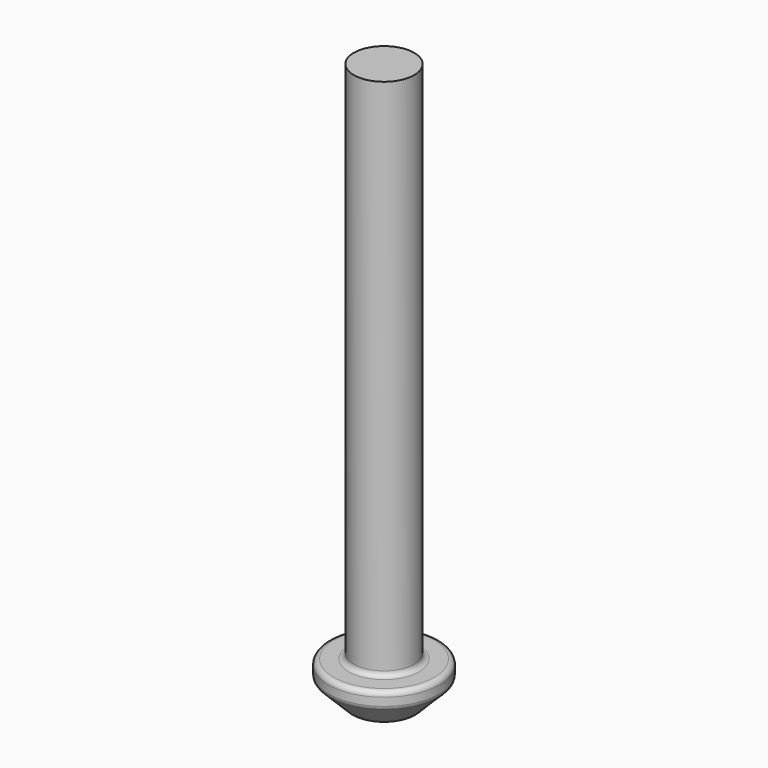
from build123d import *

# Parameters (mm, degrees)
F1_R     = 2.75
F1_R_2   = 1.5
F2_DEPTH = 2
F3_START = 1.5
F3_DEPTH = 0.5
F4_START = 2
F4_DEPTH = 26
F5_SIZE2 = 1.25
F5_SIZE  = 1.25
F6_R     = 0.25


# Not quite as in the source:
# - a feature names something its author has since deleted; it is built from what else it names


with BuildPart() as f2:
    # F1 (on Top) → F2 (new body)
    with BuildSketch(Plane.XY):
        Circle(F1_R)
        Circle(F1_R_2, mode=Mode.SUBTRACT)
        Circle(F1_R_2)
        Polygon((-0.5773502692, -1), (-1.1547005384, 0), (-0.5773502692, 1), (0.5773502692, 1), (1.1547005384, 0), (0.5773502692, -1), align=None, mode=Mode.SUBTRACT)
    extrude(amount=F2_DEPTH)

    # F1 (on Top) → F3 (join)
    with BuildSketch(Plane.XY.offset(F3_START)):
        Polygon((-0.5773502692, 1), (-1.1547005384, 0), (-0.5773502692, -1), (0.5773502692, -1), (1.1547005384, 0), (0.5773502692, 1), align=None)
    extrude(amount=F3_DEPTH)

    # F1 (on Top) → F4 (join)
    with BuildSketch(Plane.XY.offset(F4_START)):
        Circle(F1_R_2)
        Polygon((-0.5773502692, -1), (-1.1547005384, 0), (-0.5773502692, 1), (0.5773502692, 1), (1.1547005384, 0), (0.5773502692, -1), align=None, mode=Mode.SUBTRACT)
        Polygon((-0.5773502692, 1), (-1.1547005384, 0), (-0.5773502692, -1), (0.5773502692, -1), (1.1547005384, 0), (0.5773502692, 1), align=None)
    extrude(amount=F4_DEPTH)

    # F5
    f5_edges = [f2.edges().sort_by_distance(p)[0] for p in [
        (-2.75, 0, 0),
    ]]
    chamfer(f5_edges, length=F5_SIZE, length2=F5_SIZE2)

    # F6
    f6_edges = [f2.edges().sort_by_distance(p)[0] for p in [
        (-2.75, 0, 2),
        (-1.5, 0, 2),
        (-1.5, 0, 0),
        (-2.75, 0, 1.25),
    ]]
    fillet(f6_edges, radius=F6_R)


solid = f2.part
